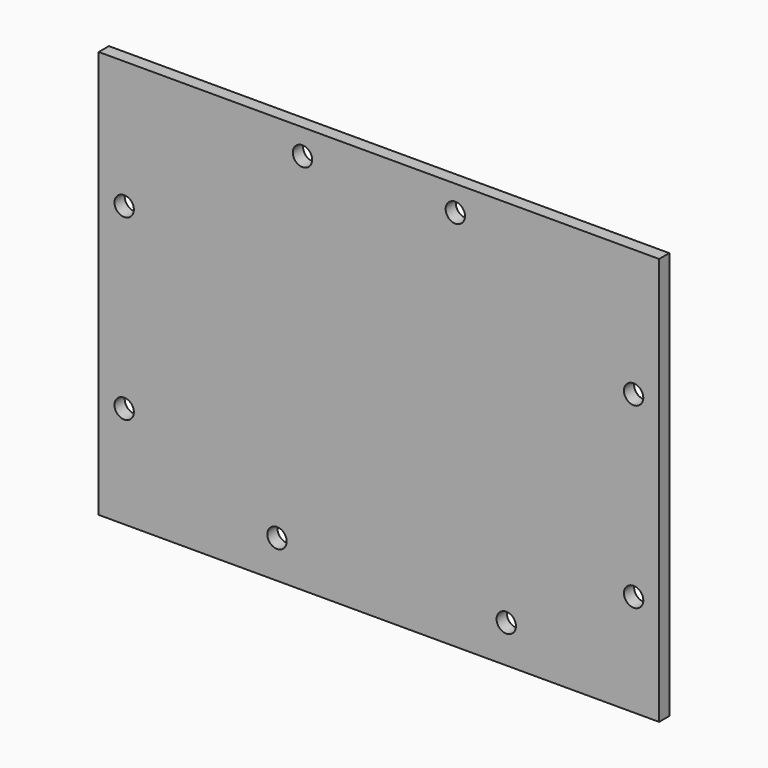
from build123d import *

# Parameters (mm, degrees)
F0_W     = 139.7
F0_H     = 101.6
F1_DEPTH = 1.5875
F2_R     = 2.413
F3_DEPTH = 3.175


# Not quite as in the source:
# - a length typed as a fraction of an inch, garbled in the dataset ("3 / 203.2 mm" for 3/8 in), is restored


with BuildPart() as f1:
    # F0 (on Front) → F1 (new body, symmetric)
    with BuildSketch(Plane.XZ):
        Rectangle(F0_W, F0_H)
    extrude(amount=F1_DEPTH, both=True)

    # F2 (on face) → F3 (cut, through all)
    with BuildSketch(Plane.XZ.offset(1.5875)):
        with Locations((-63.5, 19.05)):
            Circle(F2_R)
        with Locations((-63.5, -25.4)):
            Circle(F2_R)
        with Locations((63.5, -25.4)):
            Circle(F2_R)
        with Locations((63.5, 19.05)):
            Circle(F2_R)
        with Locations((-19.05, 44.45)):
            Circle(F2_R)
        with Locations((19.05, 44.45)):
            Circle(F2_R)
        with Locations((-25.4, -41.402)):
            Circle(F2_R)
        with Locations((31.75, -41.402)):
            Circle(F2_R)
    extrude(amount=-F3_DEPTH, mode=Mode.SUBTRACT)


solid = f1.part
